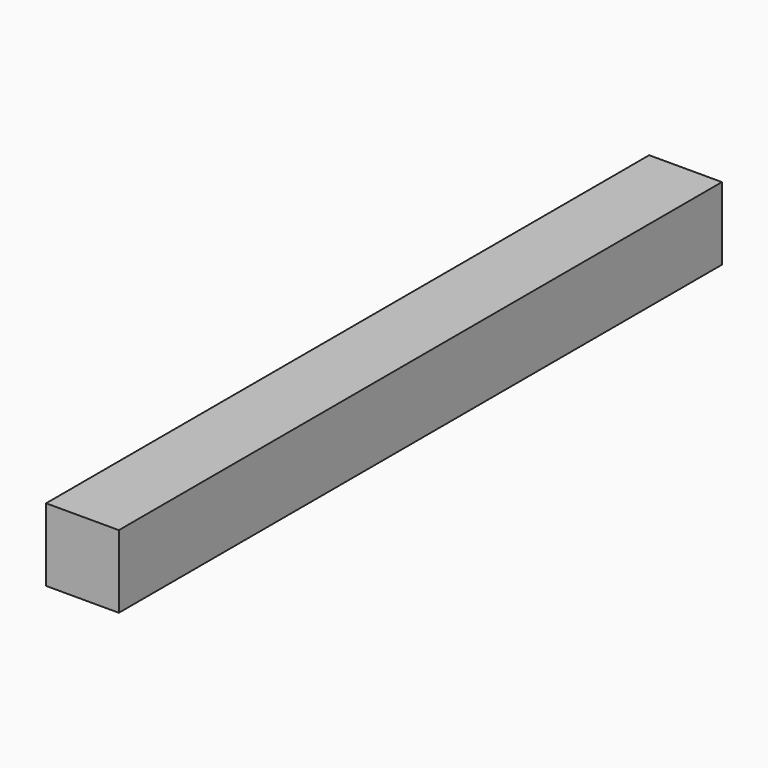
from build123d import *

# Parameters (mm, degrees)
F1_W     = 25
F1_H     = 25
F2_DEPTH = 259


with BuildPart() as f2:
    # F1 (on Front) → F2 (new body)
    with BuildSketch(Plane.XZ):
        with Locations((12.5, 12.5)):
            Rectangle(F1_W, F1_H)
    extrude(amount=F2_DEPTH)


solid = f2.part
